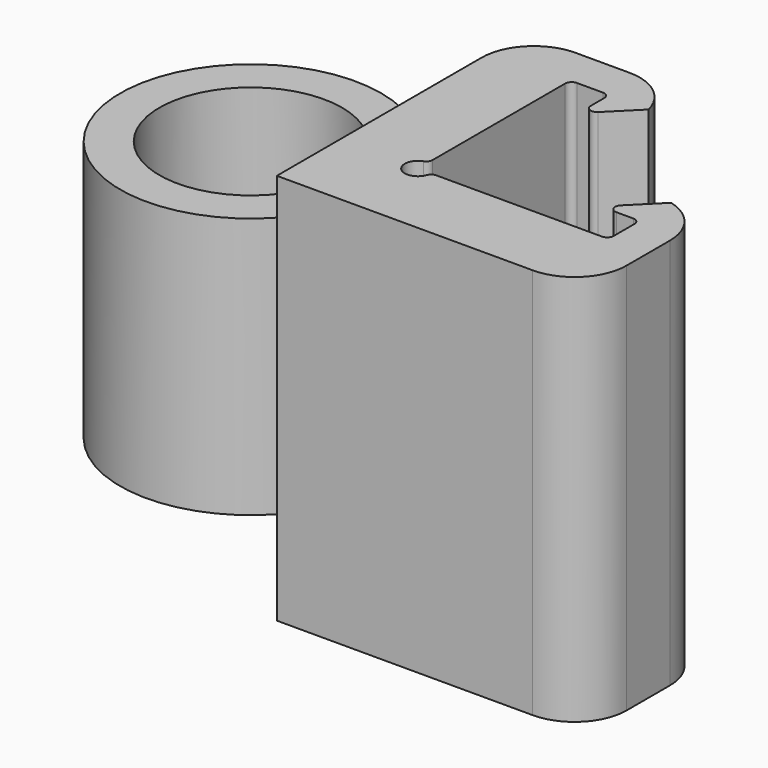
from build123d import *

# Parameters (mm, degrees)
F1_DEPTH      = 15
F2_T1_DEPTH   = 25
F2_T3_DEPTH   = 24.6824583655
F3_R          = 0.25
F6_DEPTH      = 5
F7_R          = 3.5
F8_DEPTH      = 7.501
F8_DEPTH_BACK = 7.501


# Not quite as in the source:
# - a fillet or chamfer that OpenCascade refuses, or shapes differently, is made with other operations: its cross-section is extruded or revolved along the edge and cut away or added
# - a feature names something its author has since deleted; it is built from what else it names


with BuildPart() as f1:
    # F0 (on Top) → F1 (new body)
    with BuildSketch(Plane.XY):
        with BuildLine():
            Line((3, 11.8), (0, 11.8))
            Line((0, 11.8), (0, 0))
            Line((0, 0), (11.8, 0))
            Line((11.8, 0), (11.8, 3))
            Line((11.8, 3), (11.8, 6))
            Line((11.8, 6), (10.3, 6))
            Line((10.3, 6), (8.8, 4.5))
            Line((8.8, 4.5), (10.3, 4.5))
            Line((10.3, 4.5), (10.3, 3))
            Line((10.3, 3), (3.5, 3))
            ThreePointArc((3.5, 3), (2.6464466094, 2.6464466094), (3, 3.5))
            Line((3, 3.5), (3, 10.3))
            Line((3, 10.3), (4.5, 10.3))
            Line((4.5, 10.3), (4.5, 8.8))
            Line((4.5, 8.8), (6, 10.3))
            Line((6, 10.3), (6, 11.8))
            Line((6, 11.8), (3, 11.8))
        make_face()
    extrude(amount=F1_DEPTH)

    # F2: fillet of radius 2 on 4 edges, made by hand

    # F2_s2 → F2_t1 (cut)
    with BuildSketch(Plane.XY.offset(-5)):
        with BuildLine():
            ThreePointArc((2, 11.8), (0.5857864376, 11.2142135624), (0, 9.8))
            Line((0, 9.8), (0, 11.8))
            Line((0, 11.8), (2, 11.8))
        make_face()
        with BuildLine():
            ThreePointArc((11.8, 2), (11.2142135624, 0.5857864376), (9.8, 0))
            Line((9.8, 0), (11.8, 0))
            Line((11.8, 0), (11.8, 2))
        make_face()
    extrude(amount=F2_T1_DEPTH, mode=Mode.SUBTRACT)

    # F2_s4 → F2_t3 (cut)
    with BuildSketch(Plane.XY.offset(-4.8412291828)):
        with BuildLine():
            ThreePointArc((4.0635083269, 11.8), (5.2882531983, 11.3811388301), (6, 10.3))
            Line((6, 10.3), (6, 11.8))
            Line((6, 11.8), (4.0635083269, 11.8))
        make_face()
        with BuildLine():
            ThreePointArc((10.3, 6), (11.3811388301, 5.2882531983), (11.8, 4.0635083269))
            Line((11.8, 4.0635083269), (11.8, 6))
            Line((11.8, 6), (10.3, 6))
        make_face()
    extrude(amount=F2_T3_DEPTH, mode=Mode.SUBTRACT)

    # F3
    f3_edges = [f1.edges().sort_by_distance(p)[0] for p in [
        (3, 10.3, 7.5),
        (4.5, 10.3, 7.5),
        (4.5, 8.8, 7.5),
        (3, 3.5, 7.5),
        (3.5, 3, 7.5),
        (10.3, 4.5, 7.5),
        (8.8, 4.5, 7.5),
        (10.3, 3, 7.5),
    ]]
    fillet(f3_edges, radius=F3_R)

    # F5 (on mid) → F6 (join, symmetric)
    with BuildSketch(Plane.XY.offset(7.5)):
        with BuildLine():
            ThreePointArc((-0.9090909212, 2.1252021099), (-0.2326870569, 3.4924432671), (0, 5))
            ThreePointArc((0, 5), (-0.2326870569, 6.5075567329), (-0.9090909212, 7.8747978901))
            ThreePointArc((-0.9090909212, 7.8747978901), (-10, 5), (-0.9090909212, 2.1252021099))
        make_face()
        with BuildLine():
            Line((0, 1.8377223398), (0, 5))
            ThreePointArc((0, 5), (-0.2326870569, 3.4924432671), (-0.9090909212, 2.1252021099))
            ThreePointArc((-0.9090909212, 2.1252021099), (-0.3492443377, 2.3144536376), (0, 1.8377223398))
        make_face()
        with BuildLine():
            ThreePointArc((-0.9090909212, 7.8747978901), (-0.2326870569, 6.5075567329), (0, 5))
            Line((0, 5), (0, 8.1622776602))
            ThreePointArc((0, 8.1622776602), (-0.3492443377, 7.6855463624), (-0.9090909212, 7.8747978901))
        make_face()
    extrude(amount=F6_DEPTH, both=True)

    # F7 (on mid) → F8 (cut, two sides)
    with BuildSketch(Plane.XY.offset(7.5)) as f8_sk:
        with Locations((-5, 5)):
            Circle(F7_R)
    extrude(amount=-F8_DEPTH, mode=Mode.SUBTRACT)
    extrude(f8_sk.sketch, amount=F8_DEPTH_BACK, mode=Mode.SUBTRACT)


solid = f1.part
